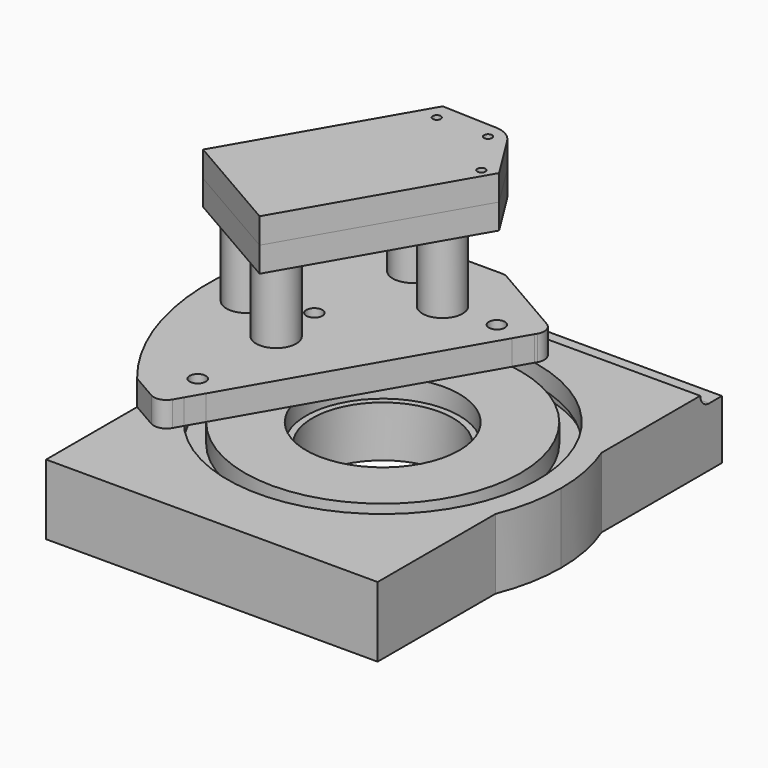
from build123d import *

# Parameters (mm, degrees)
F0_R            = 162.71875
F0_R_2          = 137.31875
F0_R_3          = 76.2
F0_R_4          = 69.85
F1_DEPTH        = 69.85
F2_START        = 50.8
F2_DEPTH        = 19.05
F4_DEPTH        = 177.801
F4_DEPTH_BACK   = 177.801
F8_DEPTH        = 25
F10_D           = 16
F13_START       = 98.4
F12_R           = 20
F12_R_2         = 8
F12_R_3         = 4
F13_DEPTH       = 25.4
F14_START       = 73.4
F14_DEPTH       = 25
F15_DEPTH       = 73.4
F17_D           = 16
F17_CBORE_D     = 32.5
F17_CBORE_DEPTH = 16
F18_D           = 6.8
F19_D           = 14
F21_DEPTH       = 25


# Not quite as in the source:
# - a feature names something its author has since deleted; it is built from what else it names


with BuildPart() as f1:
    # F0 (on Top) → F1 (new body)
    with BuildSketch(Plane.XY):
        with BuildLine():
            Line((165.1, -212.725), (165.1, -65.9911357684))
            ThreePointArc((165.1, -65.9911357684), (0, -177.8), (-165.1, -65.9911357684))
            Line((-165.1, -65.9911357684), (-165.1, -212.725))
            Line((-165.1, -212.725), (0, -212.725))
            Line((0, -212.725), (165.1, -212.725))
        make_face()
        with BuildLine():
            ThreePointArc((-165.1, 65.9911357684), (0, 177.8), (165.1, 65.9911357684))
            Line((165.1, 65.9911357684), (165.1, 215.9))
            Line((165.1, 215.9), (0, 215.9))
            Line((0, 215.9), (-165.1, 215.9))
            Line((-165.1, 215.9), (-165.1, 65.9911357684))
        make_face()
        with BuildLine():
            ThreePointArc((165.1, -65.9911357684), (174.5961339778, -33.6010416505), (177.8, 0))
            ThreePointArc((177.8, 0), (174.5961339778, 33.6010416505), (165.1, 65.9911357684))
            ThreePointArc((165.1, 65.9911357684), (0, 177.8), (-165.1, 65.9911357684))
            ThreePointArc((-165.1, 65.9911357684), (-177.8, 0), (-165.1, -65.9911357684))
            ThreePointArc((-165.1, -65.9911357684), (0, -177.8), (165.1, -65.9911357684))
        make_face()
        Circle(F0_R, mode=Mode.SUBTRACT)
        Circle(F0_R)
        Circle(F0_R_2, mode=Mode.SUBTRACT)
        Circle(F0_R_2)
        Circle(F0_R_3, mode=Mode.SUBTRACT)
        Circle(F0_R_3)
        Circle(F0_R_4, mode=Mode.SUBTRACT)
    extrude(amount=F1_DEPTH)

    # F0 (on Top) → F2 (cut)
    with BuildSketch(Plane.XY.offset(F2_START)):
        Circle(F0_R_3)
        Circle(F0_R_4, mode=Mode.SUBTRACT)
    extrude(amount=F2_DEPTH, mode=Mode.SUBTRACT)

    # F3 (on Right) → F4 (cut, two sides)
    with BuildSketch(Plane.YZ) as f4_sk:
        with BuildLine():
            Line((215.9, 58.7375), (215.9, 69.85))
            Line((215.9, 69.85), (188.9125, 69.85))
            ThreePointArc((188.9125, 69.85), (192.1672758941, 61.9922758941), (200.025, 58.7375))
            Line((200.025, 58.7375), (215.9, 58.7375))
        make_face()
    extrude(amount=-F4_DEPTH, mode=Mode.SUBTRACT)
    extrude(f4_sk.sketch, amount=F4_DEPTH_BACK, mode=Mode.SUBTRACT)

    # F3 (on Right) → F5 (revolve, cut)
    with BuildSketch(Plane.YZ):
        Polygon((154.78125, 50.8), (154.78125, 69.85), (137.31875, 69.85), (137.31875, 50.8), (132.55625, 50.8), (132.55625, 41.275), (159.54375, 41.275), (159.54375, 50.8), align=None)
    revolve(axis=Axis((0, 0, 34.925), (0, 0, 1)), mode=Mode.SUBTRACT)


with BuildPart() as f8:
    # F7 (on face) → F8 (new body)
    with BuildSketch(Plane.XY.offset(69.85)):
        with BuildLine():
            Line((-4.0562788307, 188.9125), (-50.8, 215.9))
            Line((-50.8, 215.9), (-127.7896583964, 260.35))
            ThreePointArc((-127.7896583964, 260.35), (-137.4266602692, 261.6187353658), (-145.1381810245, 255.7014773719))
            Line((-145.1381810245, 255.7014773719), (-253.0881810245, 68.7265926949))
            ThreePointArc((-253.0881810245, 68.7265926949), (-229.9227798824, -26.233366017), (-165.1, -99.3909820045))
            Line((-165.1, -99.3909820045), (-165.1, -65.9911357684))
            ThreePointArc((-165.1, -65.9911357684), (-177.8, 0), (-165.1, 65.9911357684))
            Line((-165.1, 65.9911357684), (-165.1, 188.9125))
            Line((-165.1, 188.9125), (-4.0562788307, 188.9125))
        make_face()
        with BuildLine():
            Line((26.1896583964, 171.45), (-4.0562788307, 188.9125))
            Line((-4.0562788307, 188.9125), (-165.1, 188.9125))
            Line((-165.1, 188.9125), (-165.1, 65.9911357684))
            ThreePointArc((-165.1, 65.9911357684), (-177.8, 0), (-165.1, -65.9911357684))
            Line((-165.1, -65.9911357684), (-165.1, -99.3909820045))
            Line((-165.1, -99.3909820045), (-138.9103416036, -114.5115883296))
            ThreePointArc((-138.9103416036, -114.5115883296), (-129.2733397308, -115.7803236954), (-121.5618189755, -109.8630657016))
            Line((-121.5618189755, -109.8630657016), (-116.7817522221, -101.5837472212))
            ThreePointArc((-116.7817522221, -101.5837472211), (-134.0444945295, 77.390625), (29.5832295941, 151.9278377334))
            Line((29.5832295941, 151.9278377334), (30.8381810245, 154.1014773719))
            ThreePointArc((30.8381810245, 154.1014773719), (32.1069163903, 163.7384792447), (26.1896583964, 171.45))
        make_face()
        with BuildLine():
            Line((-107.4778799044, -85.4689676597), (20.2793572763, 135.813058172))
            ThreePointArc((20.2793572763, 135.813058172), (-118.9215259159, 68.659375), (-107.4778799044, -85.4689676597))
        make_face()
        with BuildLine():
            Line((20.2793572763, 135.813058172), (29.5832295941, 151.9278377334))
            ThreePointArc((29.5832295941, 151.9278377334), (-134.0444945295, 77.390625), (-116.7817522221, -101.5837472211))
            Line((-116.7817522221, -101.5837472212), (-107.4778799044, -85.4689676597))
            ThreePointArc((-107.4778799044, -85.4689676597), (-118.9215259159, 68.659375), (20.2793572763, 135.813058172))
        make_face()
    extrude(amount=F8_DEPTH)

    # F10 (through all)
    with Locations(Plane.XY.offset(94.85)):
        with Locations((-3.1594679801, 146.015821958), (-126.4830102227, 73.025), (-128.0331451602, -70.2717314458)):
            Hole(F10_D / 2)

    # F19 (through all)
    with Locations(Plane.XY.offset(94.85)):
        with Locations((-55.6474434298, 144.0039816927), (-110.6400565702, 175.7539816927), (-125.1036934298, 23.7022277895), (-180.0963065702, 55.4522277895)):
            Hole(F19_D / 2)

    # F20 (on face) → F21 (cut, through all)
    with BuildSketch(Plane.XY.offset(94.85)):
        with BuildLine():
            Line((-205.3575752753, 151.3984269285), (-253.0881810245, 68.7265926949))
            ThreePointArc((-253.0881810245, 68.7265926949), (-229.9227798824, -26.233366017), (-165.1, -99.3909820045))
            ThreePointArc((-165.1, -99.3909820045), (-218.8281974346, 20.6102300699), (-205.3575752753, 151.3984269285))
        make_face()
        with BuildLine():
            Line((-145.1381810245, 255.7014773719), (-165.1, 221.1265926949))
            Line((-165.1, 221.1265926949), (-165.1, 215.9))
            Line((-165.1, 215.9), (-160.7852262806, 215.9))
            Line((-160.7852262806, 215.9), (-54.2029547439, 215.9))
            ThreePointArc((-54.2029547439, 215.9), (-50.9159528711, 215.4672579939), (-47.8529547439, 214.1985226281))
            Line((-47.8529547439, 214.1985226281), (-127.7896583964, 260.35))
            ThreePointArc((-127.7896583964, 260.35), (-137.4266602692, 261.6187353658), (-145.1381810245, 255.7014773719))
        make_face()
        with BuildLine():
            Line((-165.1, 221.1265926949), (-171.7837489087, 209.55))
            ThreePointArc((-171.7837489087, 209.55), (-168.9368556718, 212.9386312318), (-165.1, 215.1445689646))
            Line((-165.1, 215.1445689646), (-165.1, 215.9))
            Line((-165.1, 215.9), (-165.1, 221.1265926949))
        make_face()
        with BuildLine():
            Line((-165.1, 215.9), (-165.1, 215.1445689646))
            ThreePointArc((-165.1, 215.1445689646), (-162.9754287997, 215.7097167404), (-160.7852262806, 215.9))
            Line((-160.7852262806, 215.9), (-165.1, 215.9))
        make_face()
    extrude(amount=-F21_DEPTH, mode=Mode.SUBTRACT)


with BuildPart() as f13:
    # F12 (on face) → F13 (new body)
    with BuildSketch(Plane.XY.offset(94.85).offset(F13_START)):
        with BuildLine():
            ThreePointArc((-41.9885011187, 207.4090798685), (-45.8752843803, 212.1930996127), (-50.7999996193, 215.8999997802))
            ThreePointArc((-50.7999996193, 215.8999997802), (-56.472627292, 218.3114785178), (-62.5591019761, 219.2855218108))
            Line((-62.5591019761, 219.2855218108), (-117.3304824833, 221.3158240869))
            Line((-117.3304824833, 221.3158240869), (-217.3429824833, 48.0890926949))
            Line((-217.3429824833, 48.0890926949), (-165.1, 17.9265926949))
            Line((-165.1, 17.9265926949), (-112.8570175167, -12.2359073051))
            Line((-112.8570175167, -12.2359073051), (-12.8445175167, 160.9908240869))
            Line((-12.8445175167, 160.9908240869), (-41.9885011187, 207.4090798685))
        make_face()
        with Locations((-125.1036934298, 23.7022277895)):
            Circle(F12_R, mode=Mode.SUBTRACT)
        with Locations((-180.0963065702, 55.4522277895)):
            Circle(F12_R, mode=Mode.SUBTRACT)
        with Locations((-126.4830102227, 73.025)):
            Circle(F12_R_2, mode=Mode.SUBTRACT)
        with Locations((-110.6400565702, 175.7539816927)):
            Circle(F12_R, mode=Mode.SUBTRACT)
        with Locations((-55.6474434298, 144.0039816927)):
            Circle(F12_R, mode=Mode.SUBTRACT)
        with Locations((-26.6496594878, 156.1296167873)):
            Circle(F12_R_3, mode=Mode.SUBTRACT)
        with Locations((-109.1385791982, 203.7546167873)):
            Circle(F12_R_3, mode=Mode.SUBTRACT)
        with Locations((-57.94375, 203.5266620434)):
            Circle(F12_R_3, mode=Mode.SUBTRACT)
        with Locations((-55.6474434298, 144.0039816927)):
            Circle(F12_R)
        with Locations((-55.6474434298, 144.0039816927)):
            Circle(F12_R_2, mode=Mode.SUBTRACT)
        with Locations((-110.6400565702, 175.7539816927)):
            Circle(F12_R)
        with Locations((-110.6400565702, 175.7539816927)):
            Circle(F12_R_2, mode=Mode.SUBTRACT)
        with Locations((-125.1036934298, 23.7022277895)):
            Circle(F12_R)
        with Locations((-125.1036934298, 23.7022277895)):
            Circle(F12_R_2, mode=Mode.SUBTRACT)
        with Locations((-180.0963065702, 55.4522277895)):
            Circle(F12_R)
        with Locations((-180.0963065702, 55.4522277895)):
            Circle(F12_R_2, mode=Mode.SUBTRACT)
        with Locations((-55.6474434298, 144.0039816927)):
            Circle(F12_R_2)
        with Locations((-110.6400565702, 175.7539816927)):
            Circle(F12_R_2)
        with Locations((-125.1036934298, 23.7022277895)):
            Circle(F12_R_2)
        with Locations((-180.0963065702, 55.4522277895)):
            Circle(F12_R_2)
        with Locations((-126.4830102227, 73.025)):
            Circle(F12_R_2)
    extrude(amount=F13_DEPTH)


with BuildPart() as f14:
    # F12 (on face) → F14 (new body)
    with BuildSketch(Plane.XY.offset(94.85).offset(F14_START)):
        with BuildLine():
            ThreePointArc((-41.9885011187, 207.4090798685), (-45.8752843803, 212.1930996127), (-50.7999996193, 215.8999997802))
            ThreePointArc((-50.7999996193, 215.8999997802), (-56.472627292, 218.3114785178), (-62.5591019761, 219.2855218108))
            Line((-62.5591019761, 219.2855218108), (-117.3304824833, 221.3158240869))
            Line((-117.3304824833, 221.3158240869), (-217.3429824833, 48.0890926949))
            Line((-217.3429824833, 48.0890926949), (-165.1, 17.9265926949))
            Line((-165.1, 17.9265926949), (-112.8570175167, -12.2359073051))
            Line((-112.8570175167, -12.2359073051), (-12.8445175167, 160.9908240869))
            Line((-12.8445175167, 160.9908240869), (-41.9885011187, 207.4090798685))
        make_face()
        with Locations((-125.1036934298, 23.7022277895)):
            Circle(F12_R, mode=Mode.SUBTRACT)
        with Locations((-180.0963065702, 55.4522277895)):
            Circle(F12_R, mode=Mode.SUBTRACT)
        with Locations((-126.4830102227, 73.025)):
            Circle(F12_R_2, mode=Mode.SUBTRACT)
        with Locations((-110.6400565702, 175.7539816927)):
            Circle(F12_R, mode=Mode.SUBTRACT)
        with Locations((-55.6474434298, 144.0039816927)):
            Circle(F12_R, mode=Mode.SUBTRACT)
        with Locations((-26.6496594878, 156.1296167873)):
            Circle(F12_R_3, mode=Mode.SUBTRACT)
        with Locations((-109.1385791982, 203.7546167873)):
            Circle(F12_R_3, mode=Mode.SUBTRACT)
        with Locations((-57.94375, 203.5266620434)):
            Circle(F12_R_3, mode=Mode.SUBTRACT)
        with Locations((-55.6474434298, 144.0039816927)):
            Circle(F12_R)
        with Locations((-55.6474434298, 144.0039816927)):
            Circle(F12_R_2, mode=Mode.SUBTRACT)
        with Locations((-110.6400565702, 175.7539816927)):
            Circle(F12_R)
        with Locations((-110.6400565702, 175.7539816927)):
            Circle(F12_R_2, mode=Mode.SUBTRACT)
        with Locations((-125.1036934298, 23.7022277895)):
            Circle(F12_R)
        with Locations((-125.1036934298, 23.7022277895)):
            Circle(F12_R_2, mode=Mode.SUBTRACT)
        with Locations((-180.0963065702, 55.4522277895)):
            Circle(F12_R)
        with Locations((-180.0963065702, 55.4522277895)):
            Circle(F12_R_2, mode=Mode.SUBTRACT)
        with Locations((-55.6474434298, 144.0039816927)):
            Circle(F12_R_2)
        with Locations((-110.6400565702, 175.7539816927)):
            Circle(F12_R_2)
        with Locations((-125.1036934298, 23.7022277895)):
            Circle(F12_R_2)
        with Locations((-180.0963065702, 55.4522277895)):
            Circle(F12_R_2)
        with Locations((-126.4830102227, 73.025)):
            Circle(F12_R_2)
        with Locations((-57.94375, 203.5266620434)):
            Circle(F12_R_3)
        with Locations((-26.6496594878, 156.1296167873)):
            Circle(F12_R_3)
        with Locations((-109.1385791982, 203.7546167873)):
            Circle(F12_R_3)
    extrude(amount=F14_DEPTH)

    # F17 (through all)
    with Locations(Plane.XY.offset(193.25)):
        with Locations((-55.6474434298, 144.0039816927), (-110.6400565702, 175.7539816927), (-125.1036934298, 23.7022277895), (-180.0963065702, 55.4522277895)):
            CounterBoreHole(F17_D / 2, F17_CBORE_D / 2, F17_CBORE_DEPTH)

    # F18 (through all)
    with Locations(Plane(origin=(0, 0, 94.85), x_dir=(1, 0, 0), z_dir=(0, 0, -1))):
        with Locations((-26.6496594878, -156.1296167873), (-57.94375, -203.5266620434), (-109.1385791982, -203.7546167873)):
            Hole(F18_D / 2)


with BuildPart() as f15:
    # F12 (on face) → F15 (new body, through all)
    with BuildSketch(Plane.XY.offset(94.85)):
        with Locations((-55.6474434298, 144.0039816927)):
            Circle(F12_R)
        with Locations((-55.6474434298, 144.0039816927)):
            Circle(F12_R_2, mode=Mode.SUBTRACT)
    extrude(amount=F15_DEPTH)


with BuildPart() as f15b:
    # F12 (on face) → F15, piece 2 (new body, through all)
    with BuildSketch(Plane.XY.offset(94.85)):
        with Locations((-110.6400565702, 175.7539816927)):
            Circle(F12_R)
        with Locations((-110.6400565702, 175.7539816927)):
            Circle(F12_R_2, mode=Mode.SUBTRACT)
    extrude(amount=F15_DEPTH)


with BuildPart() as f15c:
    # F12 (on face) → F15, piece 3 (new body, through all)
    with BuildSketch(Plane.XY.offset(94.85)):
        with Locations((-180.0963065702, 55.4522277895)):
            Circle(F12_R)
        with Locations((-180.0963065702, 55.4522277895)):
            Circle(F12_R_2, mode=Mode.SUBTRACT)
    extrude(amount=F15_DEPTH)


with BuildPart() as f15d:
    # F12 (on face) → F15, piece 4 (new body, through all)
    with BuildSketch(Plane.XY.offset(94.85)):
        with Locations((-125.1036934298, 23.7022277895)):
            Circle(F12_R)
        with Locations((-125.1036934298, 23.7022277895)):
            Circle(F12_R_2, mode=Mode.SUBTRACT)
    extrude(amount=F15_DEPTH)


solid = Compound([f1.part, f8.part, f13.part, f14.part, f15.part, f15b.part, f15c.part, f15d.part])
